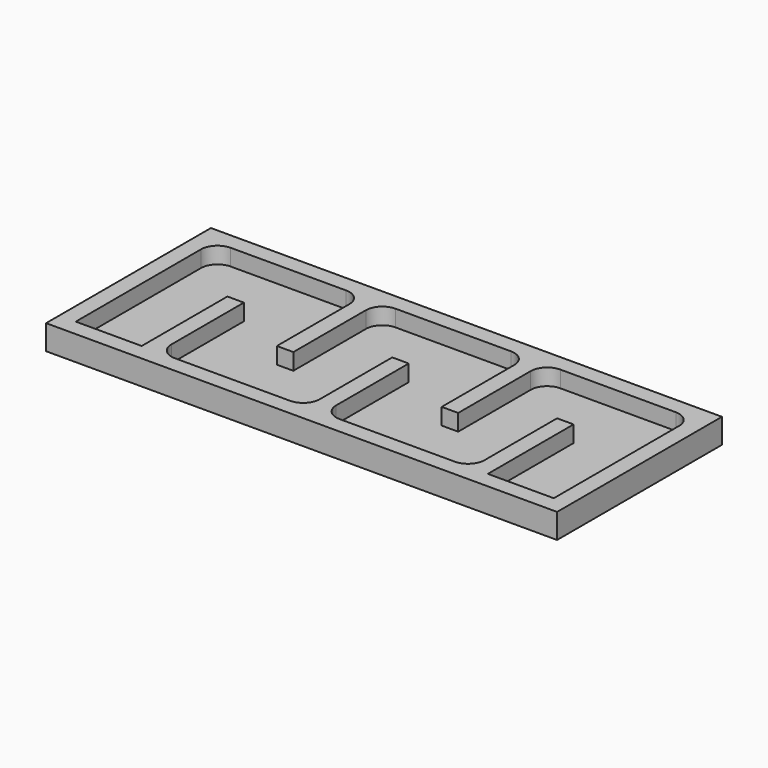
from build123d import *

# Parameters (mm, degrees)
F0_W     = 62
F0_H     = 25
F1_DEPTH = 1
F2_W     = 62
F2_H     = 25
F3_DEPTH = 2


# Not quite as in the source:
# - a feature names something its author has since deleted; it is built from what else it names


with BuildPart() as f1:
    # F0 (on Top) → F1 (new body)
    with BuildSketch(Plane.XY):
        Rectangle(F0_W, F0_H)
    extrude(amount=F1_DEPTH)

    # F2 (on face) → F3 (join)
    with BuildSketch(Plane.XY.offset(1)):
        Rectangle(F2_W, F2_H)
        with BuildLine():
            ThreePointArc((-29, 8.5), (-28.4142135624, 9.9142135624), (-27, 10.5))
            Line((-27, 10.5), (-13, 10.5))
            ThreePointArc((-13, 10.5), (-11.5857864376, 9.9142135624), (-11, 8.5))
            Line((-11, 8.5), (-11, -2.5))
            Line((-11, -2.5), (-9, -2.5))
            Line((-9, -2.5), (-9, 8.5))
            ThreePointArc((-9, 8.5), (-8.4142135624, 9.9142135624), (-7, 10.5))
            Line((-7, 10.5), (7, 10.5))
            ThreePointArc((7, 10.5), (8.4142135624, 9.9142135624), (9, 8.5))
            Line((9, 8.5), (9, -2.5))
            Line((9, -2.5), (11, -2.5))
            Line((11, -2.5), (11, 8.5))
            ThreePointArc((11, 8.5), (11.5857864376, 9.9142135624), (13, 10.5))
            Line((13, 10.5), (27, 10.5))
            ThreePointArc((27, 10.5), (28.4142135624, 9.9142135624), (29, 8.5))
            Line((29, 8.5), (29, -10.5))
            Line((29, -10.5), (21, -10.5))
            Line((21, -10.5), (21, 2.5))
            Line((21, 2.5), (19, 2.5))
            Line((19, 2.5), (19, -8.5))
            ThreePointArc((19, -8.5), (18.4142135624, -9.9142135624), (17, -10.5))
            Line((17, -10.5), (3, -10.5))
            ThreePointArc((3, -10.5), (1.5857864376, -9.9142135624), (1, -8.5))
            Line((1, -8.5), (1, 2.5))
            Line((1, 2.5), (-1, 2.5))
            Line((-1, 2.5), (-1, -8.5))
            ThreePointArc((-1, -8.5), (-1.5857864376, -9.9142135624), (-3, -10.5))
            Line((-3, -10.5), (-17, -10.5))
            ThreePointArc((-17, -10.5), (-18.4142135624, -9.9142135624), (-19, -8.5))
            Line((-19, -8.5), (-19, 2.5))
            Line((-19, 2.5), (-21, 2.5))
            Line((-21, 2.5), (-21, -10.5))
            Line((-21, -10.5), (-29, -10.5))
            Line((-29, -10.5), (-29, 8.5))
        make_face(mode=Mode.SUBTRACT)
    extrude(amount=F3_DEPTH)


solid = f1.part
